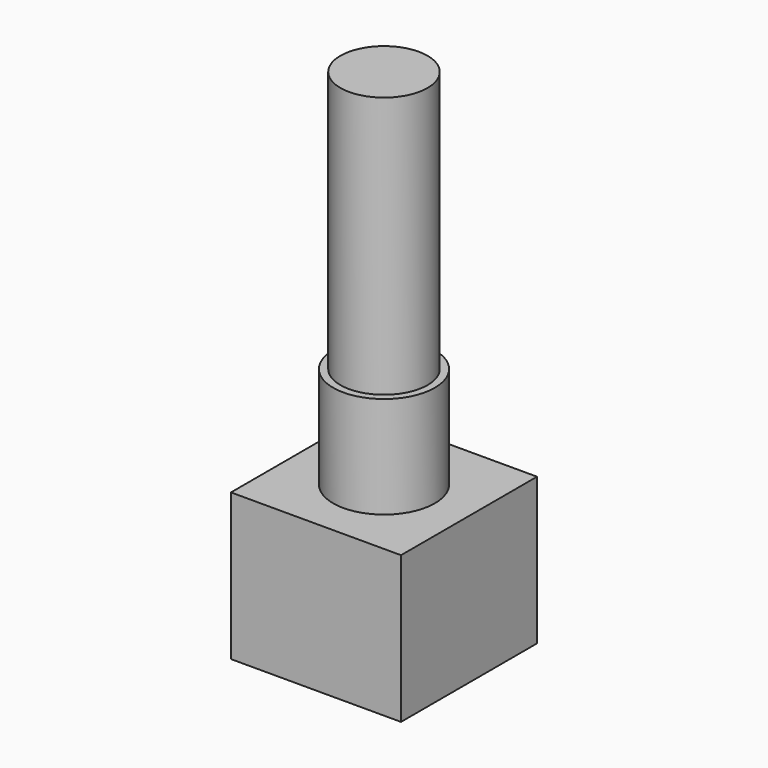
from build123d import *

# Parameters (mm, degrees)
F0_R     = 3
F1_DEPTH = 18
F2_R     = 3.5
F2_R_2   = 3
F3_DEPTH = 7
F4_W     = 11.7
F4_H     = 11.7
F4_R     = 3.5
F5_DEPTH = 10.1


with BuildPart() as f1:
    # F0 (on Top) → F1 (new body)
    with BuildSketch(Plane.XY):
        Circle(F0_R)
    extrude(amount=F1_DEPTH)

    # F2 (on face) → F3 (join)
    with BuildSketch(Plane(origin=(0, 0, 0), x_dir=(1, 0, 0), z_dir=(0, 0, -1))):
        Circle(F2_R)
        Circle(F2_R_2, mode=Mode.SUBTRACT)
        Circle(F2_R_2)
    extrude(amount=F3_DEPTH)

    # F4 (on face) → F5 (join)
    with BuildSketch(Plane(origin=(0, 0, -7), x_dir=(1, 0, 0), z_dir=(0, 0, -1))):
        Rectangle(F4_W, F4_H)
        Circle(F4_R, mode=Mode.SUBTRACT)
        Circle(F4_R)
    extrude(amount=F5_DEPTH)


solid = f1.part
